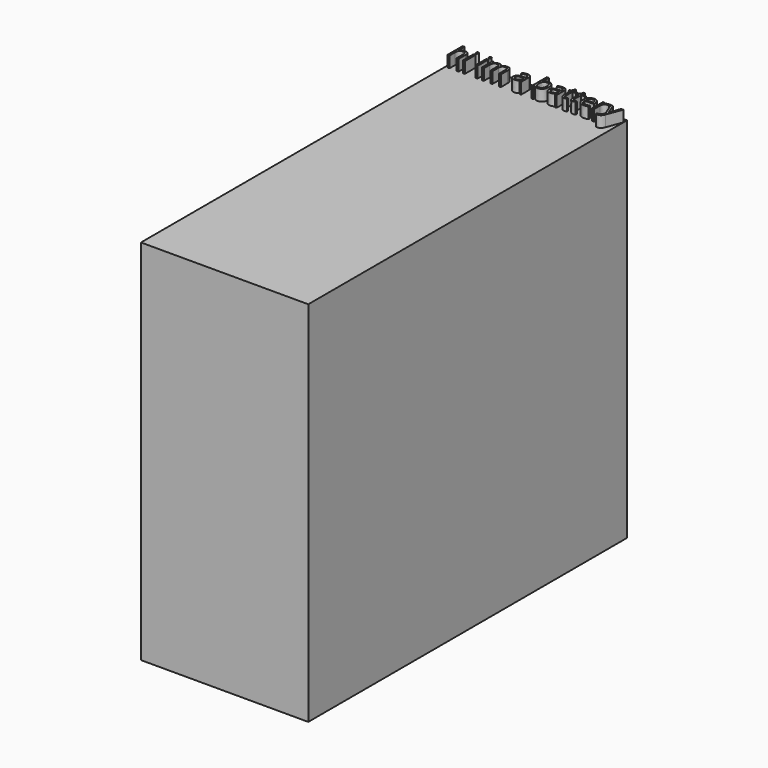
from build123d import *

# Parameters (mm, degrees)
F0_W         = 76
F0_H         = 167
F1_DEPTH     = 181
F2_TEXT_SIZE = 11.288263826
F3_DEPTH     = 5.08


# Not quite as in the source:
# - Text() gives the source's letters only with a copy of the font that has no kerning and outlines rounded to 1/6400 em; it was checked with that copy


with BuildPart() as f1:
    # F0 (on Front) → F1 (new body)
    with BuildSketch(Plane.XZ):
        with Locations((-9.057664603, 41.521659404)):
            Rectangle(F0_W, F0_H)
    extrude(amount=F1_DEPTH)

    # F2 (on face) → F3 (join)
    with BuildSketch(Plane.XY.offset(125.021659404)):
        with Locations((-47.057664603, -8.1275499547)):
            Text('hi im a battery', F2_TEXT_SIZE, font='Open Sans', text_align=(TextAlign.LEFT, TextAlign.BOTTOM))
    extrude(amount=F3_DEPTH)


solid = f1.part
